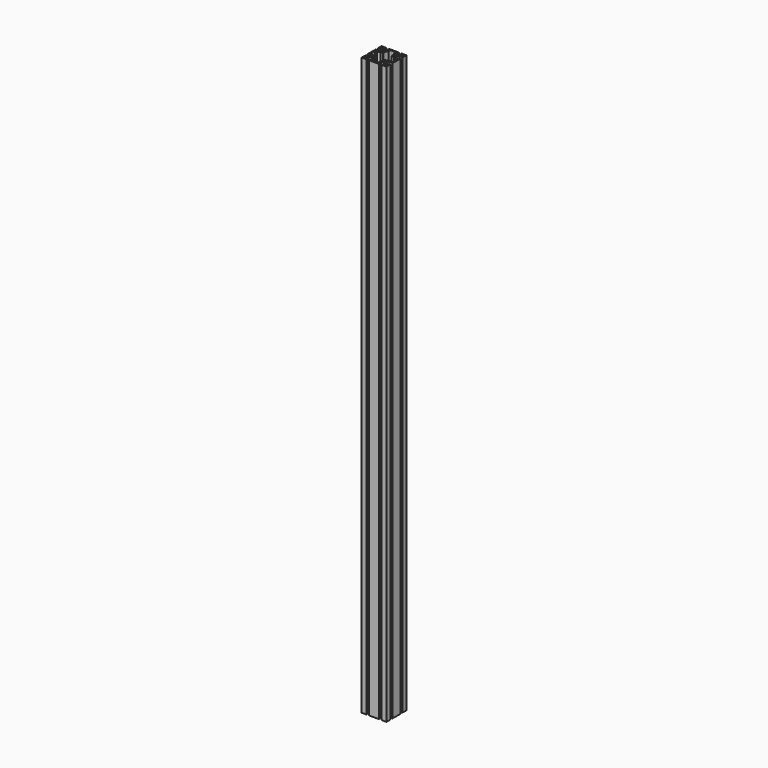
from build123d import *

# Parameters (mm, degrees)
F0_R     = 3
F0_R_2   = 2.5
F1_DEPTH = 1393
F2_R     = 2
F3_R     = 7


# Not quite as in the source:
# - a feature names something its author has since deleted; it is built from what else it names


with BuildPart() as f1:
    # F0 (on Top) → F1 (new body)
    with BuildSketch(Plane.XY):
        with BuildLine():
            Line((18.15, -30), (30, -30))
            Line((30, -30), (30, -18.15))
            Line((30, -18.15), (27.5, -18.15))
            Line((27.5, -18.15), (27.5, -20.15))
            Line((27.5, -20.15), (21.5477069044, -20.15))
            ThreePointArc((21.5477069044, -20.15), (19.5, -15), (21.5477069044, -9.85))
            Line((21.5477069044, -9.85), (27.5, -9.85))
            Line((27.5, -9.85), (27.5, -11.85))
            Line((27.5, -11.85), (30, -11.85))
            Line((30, -11.85), (30, 11.85))
            Line((30, 11.85), (27.5, 11.85))
            Line((27.5, 11.85), (27.5, 9.85))
            Line((27.5, 9.85), (21.5477069044, 9.85))
            ThreePointArc((21.5477069044, 9.85), (19.5, 15), (21.5477069044, 20.15))
            Line((21.5477069044, 20.15), (27.5, 20.15))
            Line((27.5, 20.15), (27.5, 18.15))
            Line((27.5, 18.15), (30, 18.15))
            Line((30, 18.15), (30, 30))
            Line((30, 30), (18.15, 30))
            Line((18.15, 30), (18.15, 27.5))
            Line((18.15, 27.5), (20.15, 27.5))
            Line((20.15, 27.5), (20.15, 21.5477069044))
            ThreePointArc((20.15, 21.5477069044), (15, 19.5), (9.85, 21.5477069044))
            Line((9.85, 21.5477069044), (9.85, 27.5))
            Line((9.85, 27.5), (11.85, 27.5))
            Line((11.85, 27.5), (11.85, 30))
            Line((11.85, 30), (-11.85, 30))
            Line((-11.85, 30), (-11.85, 27.5))
            Line((-11.85, 27.5), (-9.85, 27.5))
            Line((-9.85, 27.5), (-9.85, 21.5477069044))
            ThreePointArc((-9.85, 21.5477069044), (-15, 19.5), (-20.15, 21.5477069044))
            Line((-20.15, 21.5477069044), (-20.15, 27.5))
            Line((-20.15, 27.5), (-18.15, 27.5))
            Line((-18.15, 27.5), (-18.15, 30))
            Line((-18.15, 30), (-30, 30))
            Line((-30, 30), (-30, 18.15))
            Line((-30, 18.15), (-27.5, 18.15))
            Line((-27.5, 18.15), (-27.5, 20.15))
            Line((-27.5, 20.15), (-21.5477069044, 20.15))
            ThreePointArc((-21.5477069044, 20.15), (-19.5, 15), (-21.5477069044, 9.85))
            Line((-21.5477069044, 9.85), (-27.5, 9.85))
            Line((-27.5, 9.85), (-27.5, 11.85))
            Line((-27.5, 11.85), (-30, 11.85))
            Line((-30, 11.85), (-30, -11.85))
            Line((-30, -11.85), (-27.5, -11.85))
            Line((-27.5, -11.85), (-27.5, -9.85))
            Line((-27.5, -9.85), (-21.5477069044, -9.85))
            ThreePointArc((-21.5477069044, -9.85), (-19.5, -15), (-21.5477069044, -20.15))
            Line((-21.5477069044, -20.15), (-27.5, -20.15))
            Line((-27.5, -20.15), (-27.5, -18.15))
            Line((-27.5, -18.15), (-30, -18.15))
            Line((-30, -18.15), (-30, -30))
            Line((-30, -30), (-18.15, -30))
            Line((-18.15, -30), (-18.15, -27.5))
            Line((-18.15, -27.5), (-20.15, -27.5))
            Line((-20.15, -27.5), (-20.15, -21.5477069044))
            ThreePointArc((-20.15, -21.5477069044), (-15, -19.5), (-9.85, -21.5477069044))
            Line((-9.85, -21.5477069044), (-9.85, -27.5))
            Line((-9.85, -27.5), (-11.85, -27.5))
            Line((-11.85, -27.5), (-11.85, -30))
            Line((-11.85, -30), (11.85, -30))
            Line((11.85, -30), (11.85, -27.5))
            Line((11.85, -27.5), (9.85, -27.5))
            Line((9.85, -27.5), (9.85, -21.5477069044))
            ThreePointArc((9.85, -21.5477069044), (15, -19.5), (20.15, -21.5477069044))
            Line((20.15, -21.5477069044), (20.15, -27.5))
            Line((20.15, -27.5), (18.15, -27.5))
            Line((18.15, -27.5), (18.15, -30))
        make_face()
        with Locations((-25, -25)):
            Circle(F0_R, mode=Mode.SUBTRACT)
        with Locations((-15, -15)):
            Circle(F0_R_2, mode=Mode.SUBTRACT)
        with Locations((25, -25)):
            Circle(F0_R, mode=Mode.SUBTRACT)
        with Locations((15, -15)):
            Circle(F0_R_2, mode=Mode.SUBTRACT)
        with Locations((-25, 25)):
            Circle(F0_R, mode=Mode.SUBTRACT)
        with Locations((-15, 15)):
            Circle(F0_R_2, mode=Mode.SUBTRACT)
        Polygon((-7, 22), (-7, 27.5), (0, 27.5), (7, 27.5), (7, 22), (10, 16), (10, 10), (16, 10), (22, 7), (27.5, 7), (27.5, 0), (27.5, -7), (22, -7), (16, -10), (10, -10), (10, -16), (7, -22), (7, -27.5), (0, -27.5), (-7, -27.5), (-7, -22), (-10, -16), (-10, -10), (-16, -10), (-22, -7), (-27.5, -7), (-27.5, 0), (-27.5, 7), (-22, 7), (-16, 10), (-10, 10), (-10, 16), align=None, mode=Mode.SUBTRACT)
        with Locations((15, 15)):
            Circle(F0_R_2, mode=Mode.SUBTRACT)
        with Locations((25, 25)):
            Circle(F0_R, mode=Mode.SUBTRACT)
    extrude(amount=F1_DEPTH)

    # F2
    f2_edges = [f1.edges().sort_by_distance(p)[0] for p in [
        (-7, 27.5, 696.5),
        (7, 27.5, 696.5),
    ]]
    fillet(f2_edges, radius=F2_R)

    # F3
    f3_edges = [f1.edges().sort_by_distance(p)[0] for p in [
        (-10, 16, 696.5),
        (10, 16, 696.5),
    ]]
    fillet(f3_edges, radius=F3_R)


solid = f1.part
